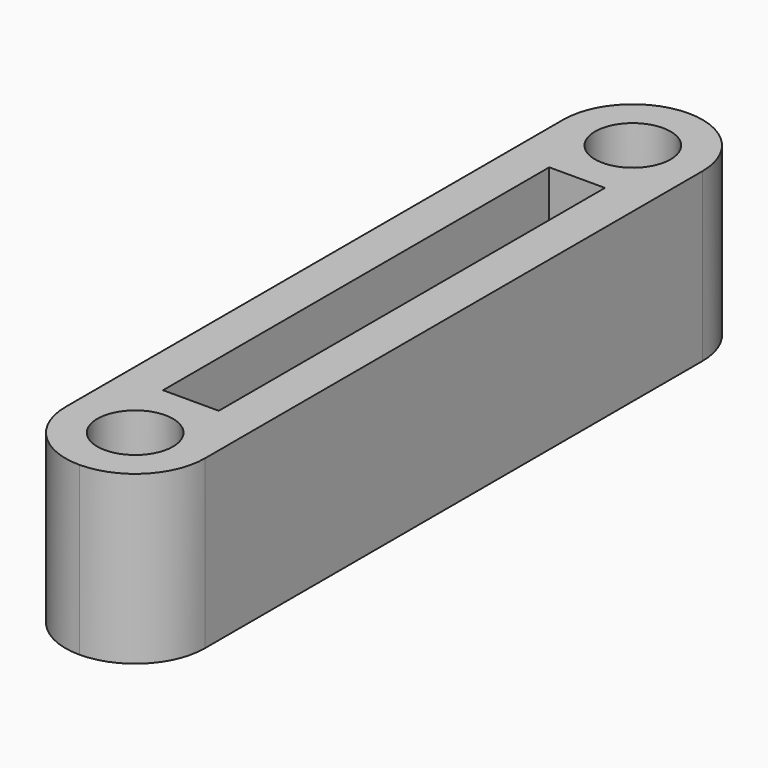
from build123d import *

# Parameters (mm, degrees)
F0_W     = 7.9375
F0_H     = 43.3812188
F0_W_2   = 3.175
F0_H_2   = 27.5062188
F1_DEPTH = 9.525
F2_R     = 2.15265
F3_DEPTH = 9.525
F4_R     = 3.96874


# Not quite as in the source:
# - a fillet or chamfer is up to 0.001 mm smaller than in the source, because OpenCascade refuses the exact size


with BuildPart() as f1:
    # F0 (on Top) → F1 (new body)
    with BuildSketch(Plane.XY):
        Rectangle(F0_W, F0_H)
        Rectangle(F0_W_2, F0_H_2, mode=Mode.SUBTRACT)
    extrude(amount=F1_DEPTH)

    # F2 (on face) → F3 (cut, through all)
    with BuildSketch(Plane.XY.offset(9.525)):
        with Locations((0, 17.7218594)):
            Circle(F2_R)
        with Locations((0, -17.7218594)):
            Circle(F2_R)
    extrude(amount=-F3_DEPTH, mode=Mode.SUBTRACT)

    # F4 (radius 3.96875 in the source; OpenCascade refuses exactly that, so slightly less here)
    f4_edges = [f1.edges().sort_by_distance(p)[0] for p in [
        (-3.96875, -21.690609, 4.7625),
        (3.96875, -21.690609, 4.7625),
        (3.96875, 21.690609, 4.7625),
        (-3.96875, 21.690609, 4.7625),
    ]]
    fillet(f4_edges, radius=F4_R)


solid = f1.part
